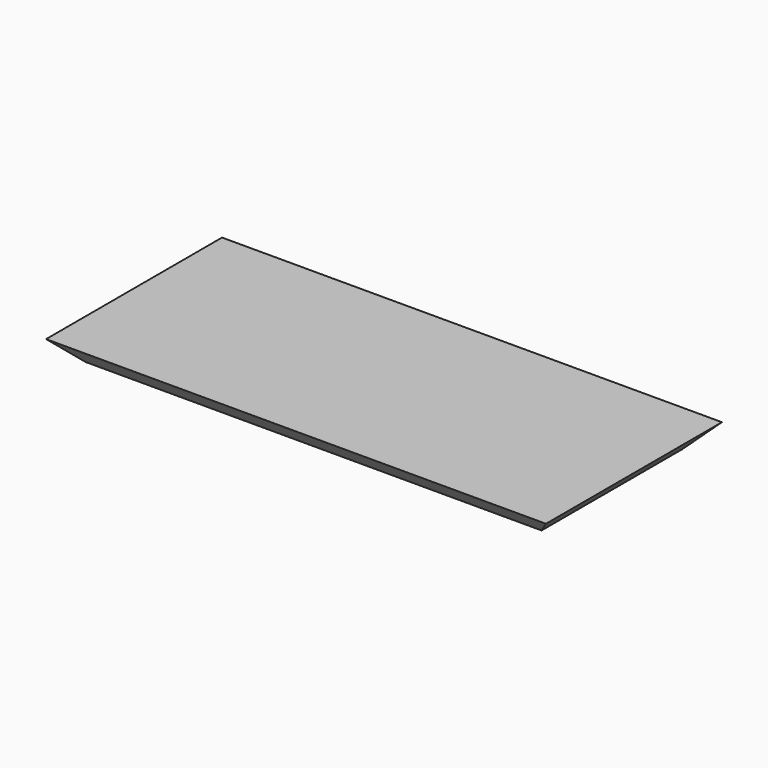
from build123d import *

# Parameters (mm, degrees)
F0_W     = 500
F0_H     = 220
F1_DEPTH = 22
F2_SIZE  = 21.99999


# Not quite as in the source:
# - a fillet or chamfer is up to 0.001 mm smaller than in the source, because OpenCascade refuses the exact size


with BuildPart() as f1:
    # F0 (on Top) → F1 (new body)
    with BuildSketch(Plane.XY):
        Rectangle(F0_W, F0_H)
    extrude(amount=F1_DEPTH)

    # F2 (size 22 in the source; OpenCascade refuses exactly that, so slightly less here)
    f2_edges = [f1.edges().sort_by_distance(p)[0] for p in [
        (0, -110, 0),
        (250, 0, 0),
        (0, 110, 0),
        (-250, 0, 0),
    ]]
    chamfer(f2_edges, length=F2_SIZE)


solid = f1.part
